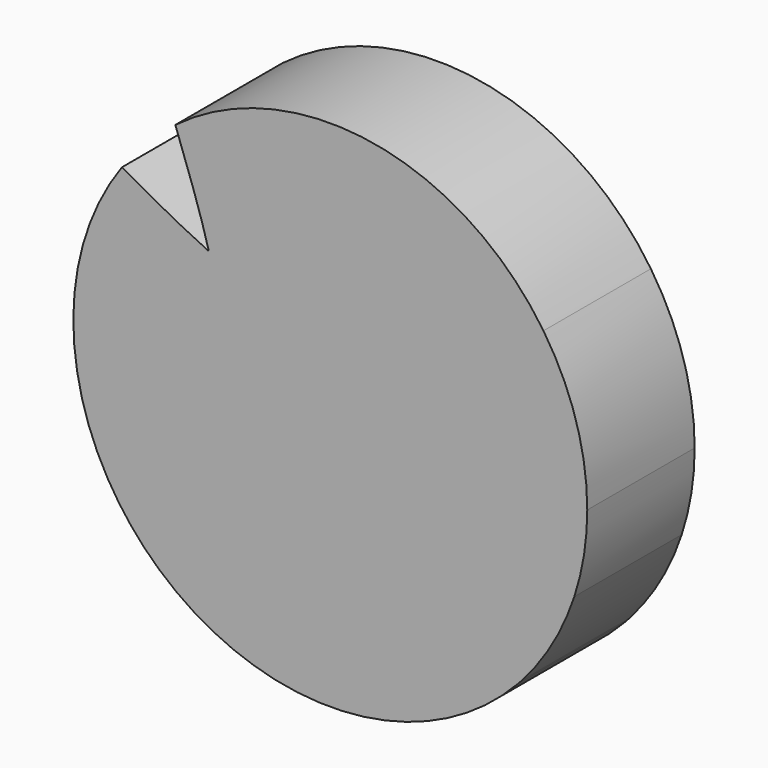
from build123d import *

# Parameters (mm, degrees)
F1_DEPTH = 25.4


with BuildPart() as f1:
    # F0 (on Front) → F1 (new body)
    with BuildSketch(Plane.XZ):
        with BuildLine():
            ThreePointArc((46.1673500078, -15.2324506451), (47.999444804, -7.7139521587), (48.6153448964, 0))
            ThreePointArc((48.6153448964, 0), (46.4980117159, 14.1910769804), (40.3304436459, 27.1460323938))
            add(Edge.make_bspline(
                [(40.3304436459, 27.1460323938), (32.3786976376, 23.0993060038), (24.4227156617, 19.0482632148), (16.5014874139, 16.4513327342)],
                knots=[0, 0, 0, 0, 0.2953409121, 0.2953409121, 0.2953409121, 0.2953409121], degree=3))
            add(Edge.make_bspline(
                [(16.5014873898, 16.4513327474), (15.5953694896, 11.2931775522), (15.5320066906, 3.0058951007), (18.67748395, -6.2871122776), (19.9799499764, -9.4342211392)],
                knots=[0.2963486373, 0.2963486373, 0.2963486373, 0.2963486373, 0.4715656378, 0.5637333, 0.5637333, 0.5637333, 0.5637333], degree=3))
            add(Edge.make_bspline(
                [(46.1673500078, -15.2324506451), (37.3947505843, -12.9712227578), (28.6158550244, -10.7067465721), (19.9799499764, -9.4342211392)],
                knots=[0, 0, 0, 0, 0.282903213, 0.282903213, 0.282903213, 0.282903213], degree=3))
        make_face()
        with BuildLine():
            add(Edge.make_bspline(
                [(40.3304436459, 27.1460323938), (32.3786976376, 23.0993060038), (24.4227156617, 19.0482632148), (16.5014874139, 16.4513327342)],
                knots=[0, 0, 0, 0, 0.2953409121, 0.2953409121, 0.2953409121, 0.2953409121], degree=3))
            ThreePointArc((40.3304436459, 27.1460323938), (33.903902399, 34.84217504), (26.0352353751, 41.056281838))
            add(Edge.make_bspline(
                [(26.0352353751, 41.056281838), (22.0398072792, 33.1200566973), (18.0340259226, 25.1754420421), (16.5014873898, 16.4513327474)],
                knots=[0, 0, 0, 0, 0.2963486373, 0.2963486373, 0.2963486373, 0.2963486373], degree=3))
        make_face()
        with BuildLine():
            ThreePointArc((36.2646535731, -32.3778730095), (42.0981018646, -24.3146371306), (46.1673500078, -15.2324506451))
            add(Edge.make_bspline(
                [(46.1673500078, -15.2324506451), (37.3947505843, -12.9712227578), (28.6158550244, -10.7067465721), (19.9799499764, -9.4342211392)],
                knots=[0, 0, 0, 0, 0.282903213, 0.282903213, 0.282903213, 0.282903213], degree=3))
            add(Edge.make_bspline(
                [(19.9799499764, -9.4342211392), (25.0191791568, -21.6103566301), (33.3249337281, -32.9452793274), (35.454034531, -33.2635415263)],
                knots=[0.5637333, 0.5637333, 0.5637333, 0.5637333, 0.9203291446, 0.9203291446, 0.9203291446, 0.9203291446], degree=3))
            ThreePointArc((35.454034531, -33.2635415263), (35.8620782725, -32.823209797), (36.2646535731, -32.3778730095))
        make_face()
        with BuildLine():
            add(Edge.make_bspline(
                [(26.0352353751, 41.056281838), (22.0398072792, 33.1200566973), (18.0340259226, 25.1754420421), (16.5014873898, 16.4513327474)],
                knots=[0, 0, 0, 0, 0.2963486373, 0.2963486373, 0.2963486373, 0.2963486373], degree=3))
            ThreePointArc((26.0352353751, 41.056281838), (-1.9947078477, 48.5744058121), (-29.3138505417, 38.7833717695))
            add(Edge.make_bspline(
                [(-29.3138505417, 38.7833717695), (-27.000307279, 32.4407823134), (-24.6802191732, 26.0937743503), (-22.973223534, 19.7963497545)],
                knots=[0, 0, 0, 0, 0.2452233004, 0.2452233004, 0.2452233004, 0.2452233004], degree=3))
            add(Edge.make_bspline(
                [(16.5014874139, 16.4513327342), (10.9797013124, 14.6410459723), (-2.2734109483, 11.9838999083), (-15.3520884673, 16.285685391), (-22.973223534, 19.7963497545)],
                knots=[0.2953409121, 0.2953409121, 0.2953409121, 0.2953409121, 0.5012192547, 0.7909956335, 0.7909956335, 0.7909956335, 0.7909956335], degree=3))
        make_face()
        with BuildLine():
            add(Edge.make_bspline(
                [(16.5014873898, 16.4513327474), (15.5953694896, 11.2931775522), (15.5320066906, 3.0058951007), (18.67748395, -6.2871122776), (19.9799499764, -9.4342211392)],
                knots=[0.2963486373, 0.2963486373, 0.2963486373, 0.2963486373, 0.4715656378, 0.5637333, 0.5637333, 0.5637333, 0.5637333], degree=3))
            add(Edge.make_bspline(
                [(16.5014874139, 16.4513327342), (10.9797013124, 14.6410459723), (-2.2734109483, 11.9838999083), (-15.3520884673, 16.285685391), (-22.973223534, 19.7963497545)],
                knots=[0.2953409121, 0.2953409121, 0.2953409121, 0.2953409121, 0.5012192547, 0.7909956335, 0.7909956335, 0.7909956335, 0.7909956335], degree=3))
            add(Edge.make_bspline(
                [(-22.973223534, 19.7963497545), (-21.1636232806, 13.1203976417), (-19.1493739324, 1.2205893586), (-21.7464907751, -10.2913075482), (-23.4240943414, -15.3533007473)],
                knots=[0.2452233004, 0.2452233004, 0.2452233004, 0.2452233004, 0.5051865577, 0.7125051709, 0.7125051709, 0.7125051709, 0.7125051709], degree=3))
            add(Edge.make_bspline(
                [(19.9799499764, -9.4342211392), (13.2080472289, -8.4363618033), (-1.6767781675, -7.5725154611), (-15.7685768428, -12.1133609217), (-23.4240943551, -15.3533007369)],
                knots=[0.282903213, 0.282903213, 0.282903213, 0.282903213, 0.5047436611, 0.776928854, 0.776928854, 0.776928854, 0.776928854], degree=3))
        make_face()
        with BuildLine():
            add(Edge.make_bspline(
                [(19.9799499764, -9.4342211392), (25.0191791568, -21.6103566301), (33.3249337281, -32.9452793274), (35.454034531, -33.2635415263)],
                knots=[0.5637333, 0.5637333, 0.5637333, 0.5637333, 0.9203291446, 0.9203291446, 0.9203291446, 0.9203291446], degree=3))
            add(Edge.make_bspline(
                [(19.9799499764, -9.4342211392), (13.2080472289, -8.4363618033), (-1.6767781675, -7.5725154611), (-15.7685768428, -12.1133609217), (-23.4240943551, -15.3533007369)],
                knots=[0.282903213, 0.282903213, 0.282903213, 0.282903213, 0.5047436611, 0.776928854, 0.776928854, 0.776928854, 0.776928854], degree=3))
            add(Edge.make_bspline(
                [(-23.4240943414, -15.3533007473), (-25.7504766345, -22.3729158592), (-29.0871025112, -29.3050684982), (-32.4143035176, -36.2320947071)],
                knots=[0.7125051709, 0.7125051709, 0.7125051709, 0.7125051709, 1, 1, 1, 1], degree=3))
            ThreePointArc((-32.4143035176, -36.2320947071), (2.1243983043, -48.5689066301), (35.454034531, -33.2635415263))
        make_face()
        with BuildLine():
            add(Edge.make_bspline(
                [(-22.973223534, 19.7963497545), (-21.1636232806, 13.1203976417), (-19.1493739324, 1.2205893586), (-21.7464907751, -10.2913075482), (-23.4240943414, -15.3533007473)],
                knots=[0.2452233004, 0.2452233004, 0.2452233004, 0.2452233004, 0.5051865577, 0.7125051709, 0.7125051709, 0.7125051709, 0.7125051709], degree=3))
            add(Edge.make_bspline(
                [(-22.973223534, 19.7963497545), (-28.4700501333, 22.3284546294), (-33.9538200156, 25.3785378793), (-39.4374864795, 28.4277403178)],
                knots=[0.7909956335, 0.7909956335, 0.7909956335, 0.7909956335, 1, 1, 1, 1], degree=3))
            ThreePointArc((-39.4374864795, 28.4277403178), (-48.5534662677, 2.4520752004), (-42.1008703821, -24.3098431189))
            add(Edge.make_bspline(
                [(-23.4240943551, -15.3533007369), (-29.6982235487, -18.0086144957), (-35.899537129, -21.1597200741), (-42.1008703821, -24.3098431189)],
                knots=[0.776928854, 0.776928854, 0.776928854, 0.776928854, 1, 1, 1, 1], degree=3))
        make_face()
        with BuildLine():
            add(Edge.make_bspline(
                [(-23.4240943414, -15.3533007473), (-25.7504766345, -22.3729158592), (-29.0871025112, -29.3050684982), (-32.4143035176, -36.2320947071)],
                knots=[0.7125051709, 0.7125051709, 0.7125051709, 0.7125051709, 1, 1, 1, 1], degree=3))
            add(Edge.make_bspline(
                [(-23.4240943551, -15.3533007369), (-29.6982235487, -18.0086144957), (-35.899537129, -21.1597200741), (-42.1008703821, -24.3098431189)],
                knots=[0.776928854, 0.776928854, 0.776928854, 0.776928854, 1, 1, 1, 1], degree=3))
            ThreePointArc((-42.1008703821, -24.3098431189), (-37.731456453, -30.6559774487), (-32.4143035176, -36.2320947071))
        make_face()
    extrude(amount=F1_DEPTH)


solid = f1.part
